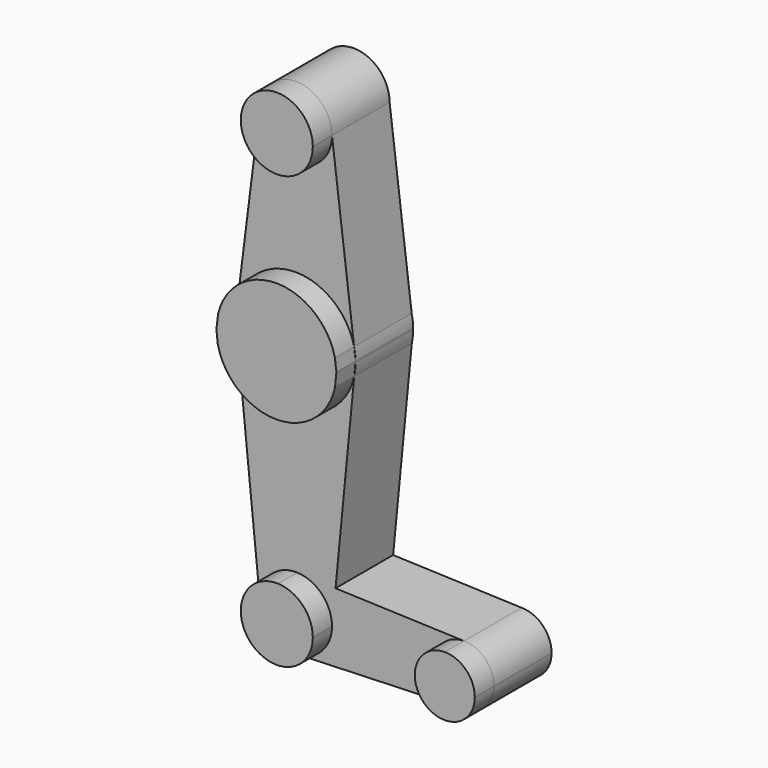
from build123d import *

# Parameters (mm, degrees)
F1_DEPTH = 25.4
F2_DEPTH = 19.05


with BuildPart() as f1:
    # F0 (on Front) → F1 (new body)
    with BuildSketch(Plane.XZ):
        with BuildLine():
            ThreePointArc((-9.4505353604, 41.5638555321), (-0.5955147738, 30.8687904621), (9.525, 40.3751560744))
            ThreePointArc((9.525, 40.3751560744), (9.5249820462, 40.3936498602), (9.5249281848, 40.4121435763))
            ThreePointArc((9.5249281848, 40.4121435763), (0.5770560461, 49.8826600223), (-9.4505353604, 41.5638555321))
        make_face()
    extrude(amount=F1_DEPTH)


with BuildPart() as f1b:
    # F0 (on Front) → F1, piece 2 (new body)
    with BuildSketch(Plane.XZ):
        with BuildLine():
            Line((15.7660711788, -10.0846397195), (15.371304716, -6.8906035395))
            ThreePointArc((15.371304716, -6.8906035395), (0.0606968294, 5.4492883552), (-15.5045872563, -6.5677652421))
            Line((-15.5045872563, -6.5677652421), (-15.9800981954, -10.3482270861))
            Line((-15.9800981954, -10.3482270861), (-15.6456242534, -13.6672845653))
            ThreePointArc((-15.6456242534, -13.6672845653), (-0.1786997991, -26.2996741605), (15.4044031981, -13.810882388))
            Line((15.4044031981, -13.810882388), (15.7660711788, -10.0846397195))
        make_face()
    extrude(amount=F1_DEPTH)


with BuildPart() as f1c:
    # F0 (on Front) → F1, piece 3 (new body)
    with BuildSketch(Plane.XZ):
        with BuildLine():
            ThreePointArc((0.3412708989, -64.4059595806), (-6.9491816059, -67.4106670775), (-9.4770004124, -74.8798770055))
            ThreePointArc((-9.4770004124, -74.8798770055), (-6.3886201528, -80.989626834), (0, -83.4498439256))
            Line((0, -83.4498439256), (0.6773435479, -83.4257297116))
            ThreePointArc((0.6773435479, -83.4257297116), (6.9705567315, -80.4161430139), (9.525, -73.9248439256))
            ThreePointArc((9.525, -73.9248439256), (6.8547877543, -67.3114098824), (0.3412708989, -64.4059595806))
        make_face()
    extrude(amount=F1_DEPTH)


with BuildPart() as f1d:
    # F0 (on Front) → F1, piece 4 (new body)
    with BuildSketch(Plane.XZ):
        with BuildLine():
            ThreePointArc((52.3875, -73.9248439256), (50.0626600757, -68.31218385), (44.45, -65.9873439256))
            ThreePointArc((44.45, -65.9873439256), (36.5137564458, -74.0660689178), (44.7324052746, -81.8573185402))
            ThreePointArc((44.7324052746, -81.8573185402), (50.1616327839, -79.4367544104), (52.3875, -73.9248439256))
        make_face()
    extrude(amount=F1_DEPTH)


with BuildPart() as f2:
    # F0 (on Front) → F2 (new body)
    with BuildSketch(Plane.XZ):
        with BuildLine():
            ThreePointArc((-9.4505353604, 41.5638555321), (-0.5955147738, 30.8687904621), (9.525, 40.3751560744))
            ThreePointArc((9.525, 40.3751560744), (9.5249820462, 40.3936498602), (9.5249281848, 40.4121435763))
            ThreePointArc((9.5249281848, 40.4121435763), (0.5770560461, 49.8826600223), (-9.4505353604, 41.5638555321))
        make_face()
        with BuildLine():
            ThreePointArc((9.5249281848, 40.4121435763), (9.5249820462, 40.3936498602), (9.525, 40.3751560744))
            ThreePointArc((9.525, 40.3751560744), (-0.5955147738, 30.8687904621), (-9.4505353604, 41.5638555321))
            Line((-9.4505353604, 41.5638555321), (-15.5045872563, -6.5677652421))
            ThreePointArc((-15.5045872563, -6.5677652421), (0.0606968294, 5.4492883552), (15.371304716, -6.8906035395))
            Line((15.371304716, -6.8906035395), (9.5249281848, 40.4121435763))
        make_face()
        with BuildLine():
            Line((15.7660711788, -10.0846397195), (15.371304716, -6.8906035395))
            ThreePointArc((15.371304716, -6.8906035395), (0.0606968294, 5.4492883552), (-15.5045872563, -6.5677652421))
            Line((-15.5045872563, -6.5677652421), (-15.9800981954, -10.3482270861))
            Line((-15.9800981954, -10.3482270861), (-15.6456242534, -13.6672845653))
            ThreePointArc((-15.6456242534, -13.6672845653), (-0.1786997991, -26.2996741605), (15.4044031981, -13.810882388))
            Line((15.4044031981, -13.810882388), (15.7660711788, -10.0846397195))
        make_face()
        with BuildLine():
            ThreePointArc((15.7660711788, -10.0846397195), (15.6498378192, -8.4775919222), (15.371304716, -6.8906035395))
            Line((15.371304716, -6.8906035395), (15.7660711788, -10.0846397195))
        make_face()
        with BuildLine():
            Line((-15.9800981954, -10.3482270861), (-15.5045872563, -6.5677652421))
            ThreePointArc((-15.5045872563, -6.5677652421), (-15.8561753502, -8.4436781627), (-15.9800981954, -10.3482270861))
        make_face()
        with BuildLine():
            ThreePointArc((15.7697169172, -10.4248439256), (15.7688054564, -10.2547320556), (15.7660711788, -10.0846397195))
            Line((15.7660711788, -10.0846397195), (15.4044031981, -13.810882388))
            ThreePointArc((15.4044031981, -13.810882388), (15.6781242602, -12.127687913), (15.7697169172, -10.4248439256))
        make_face()
        with BuildLine():
            Line((-15.6456242534, -13.6672845653), (-15.9800981954, -10.3482270861))
            ThreePointArc((-15.9800981954, -10.3482270861), (-15.9002837701, -12.0165657254), (-15.6456242534, -13.6672845653))
        make_face()
        with BuildLine():
            Line((10.4584548085, -64.7686804428), (15.4044031981, -13.810882388))
            ThreePointArc((15.4044031981, -13.810882388), (-0.1786997991, -26.2996741605), (-15.6456242534, -13.6672845653))
            Line((-15.6456242534, -13.6672845653), (-9.4770004124, -74.8798770055))
            ThreePointArc((-9.4770004124, -74.8798770055), (-6.9491816059, -67.4106670775), (0.3412708989, -64.4059595806))
            Line((0.3412708989, -64.4059595806), (10.4584548085, -64.7686804428))
        make_face()
        with BuildLine():
            Line((44.45, -65.9873439256), (10.4584548085, -64.7686804428))
            Line((10.4584548085, -64.7686804428), (0.3412708989, -64.4059595806))
            ThreePointArc((0.3412708989, -64.4059595806), (6.8547877543, -67.3114098824), (9.525, -73.9248439256))
            ThreePointArc((9.525, -73.9248439256), (6.9705567315, -80.4161430139), (0.6773435479, -83.4257297116))
            Line((0.6773435479, -83.4257297116), (44.7324052746, -81.8573185402))
            ThreePointArc((44.7324052746, -81.8573185402), (36.5137564458, -74.0660689178), (44.45, -65.9873439256))
        make_face()
        with BuildLine():
            ThreePointArc((0.3412708989, -64.4059595806), (-6.9491816059, -67.4106670775), (-9.4770004124, -74.8798770055))
            ThreePointArc((-9.4770004124, -74.8798770055), (-6.3886201528, -80.989626834), (0, -83.4498439256))
            Line((0, -83.4498439256), (0.6773435479, -83.4257297116))
            ThreePointArc((0.6773435479, -83.4257297116), (6.9705567315, -80.4161430139), (9.525, -73.9248439256))
            ThreePointArc((9.525, -73.9248439256), (6.8547877543, -67.3114098824), (0.3412708989, -64.4059595806))
        make_face()
        with BuildLine():
            ThreePointArc((52.3875, -73.9248439256), (50.0626600757, -68.31218385), (44.45, -65.9873439256))
            ThreePointArc((44.45, -65.9873439256), (36.5137564458, -74.0660689178), (44.7324052746, -81.8573185402))
            ThreePointArc((44.7324052746, -81.8573185402), (50.1616327839, -79.4367544104), (52.3875, -73.9248439256))
        make_face()
        with BuildLine():
            Line((0.6773435479, -83.4257297116), (0, -83.4498439256))
            ThreePointArc((0, -83.4498439256), (0.3388863295, -83.4438134631), (0.6773435479, -83.4257297116))
        make_face()
    extrude(amount=F2_DEPTH)


solid = Compound([f1.part, f1b.part, f1c.part, f1d.part, f2.part])
